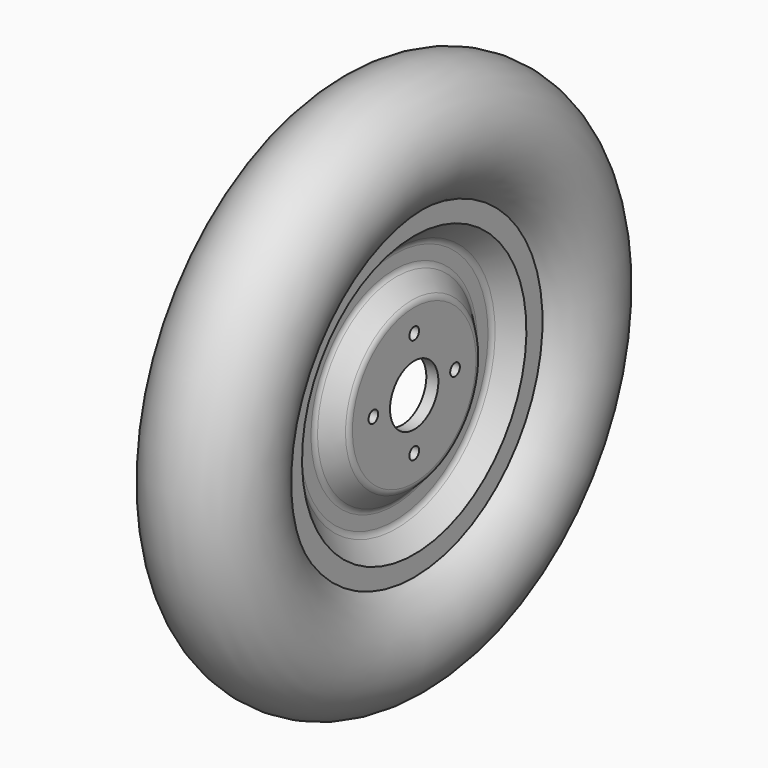
from build123d import *

# Parameters (mm, degrees)
F2_R  = 2
F4_R  = 1.9
F5_D  = 15
F7_D  = 3
F9_D  = 3
F11_D = 3
F12_R = 1.8


# Not quite as in the source:
# - a feature names something its author has since deleted; it is built from what else it names


with BuildPart() as f1:
    # F0 (on Front) → F1 (revolve)
    with BuildSketch(Plane.XZ):
        with BuildLine():
            Line((-28.4126295149, 14.8122454338), (-28.4126295149, 19.8122454338))
            ThreePointArc((-28.4126295149, 19.8122454338), (-35.9126295149, 47.8026264906), (-43.4126295149, 19.8122454338))
            Line((-43.4126295149, 19.8122454338), (-43.4126295149, 12))
            Line((-43.4126295149, 12), (-31.4126295149, 0))
            Line((-31.4126295149, 0), (-31.4126295149, -1.8659040798))
            Line((-31.4126295149, -1.8659040798), (-31.4126295149, -20))
            Line((-31.4126295149, -20), (-28.4126295149, -20))
            Line((-28.4126295149, -20), (-28.4126295149, 0))
            Line((-28.4126295149, 0), (-33.4126295149, 5))
            Line((-33.4126295149, 5), (-33.4126295149, 10))
            Line((-33.4126295149, 10), (-28.4126295149, 14.8122454338))
        make_face()
    revolve(axis=Axis((-29.9126295149, 0, -20), (-1, 0, 0)))

    # F2
    f2_edges = [f1.edges().sort_by_distance(p)[0] for p in [
        (-33.41263, 0, -50),
        (-28.41263, 0, -40),
    ]]
    fillet(f2_edges, radius=F2_R)

    # F4
    f4_edges = [f1.edges().sort_by_distance(p)[0] for p in [
        (-33.41263, 0, -45),
    ]]
    fillet(f4_edges, radius=F4_R)

    # F5 (through all)
    with Locations(Plane.YZ.offset(-28.4126295149)):
        with Locations((0, -20)):
            Hole(F5_D / 2)

    # F7 (through all)
    with Locations(Plane.YZ):
        with Locations((0, -6.5), (-12.6833414137, -19.5598490536)):
            Hole(F7_D / 2)

    # F9 (through all)
    with Locations(Plane.YZ.offset(-28.4126295149)):
        with Locations((0, -32.6715728753)):
            Hole(F9_D / 2)

    # F11 (through all)
    with Locations(Plane.YZ.offset(-28.4126295149)):
        with Locations((12.666519602, -19.5598490536)):
            Hole(F11_D / 2)

    # F12
    f12_edges = [f1.edges().sort_by_distance(p)[0] for p in [
        (-31.41263, 0, -40),
    ]]
    fillet(f12_edges, radius=F12_R)


solid = f1.part
